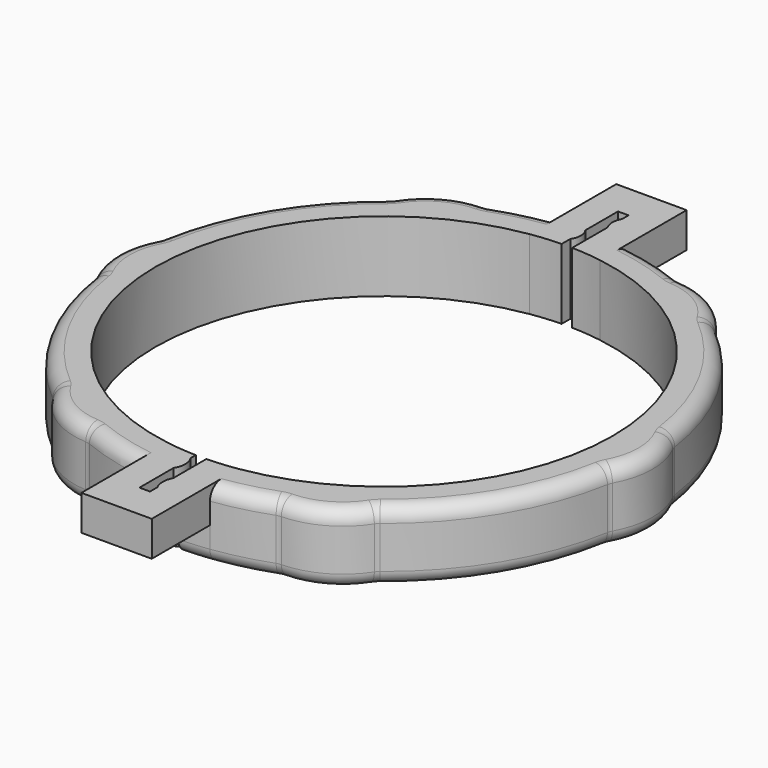
from build123d import *

# Parameters (mm, degrees)
F1_DEPTH = 10
F2_DEPTH = 5
F6_R     = 2


# Not quite as in the source:
# - a feature of the source that left no trace in its solid (it failed there, or was rolled back) is left out
# - the program builds the solid bodies; features that only make, move or delete a surface that nothing else refers to are left out


with BuildPart() as f1:
    # F0 (on Top) → F1 (new body)
    with BuildSketch(Plane.XY):
        with BuildLine():
            ThreePointArc((36.9932073794, -6.1443150788), (37.3730870863, -3.0825900858), (37.5, 0))
            ThreePointArc((37.5, 0), (37.4200494969, 2.4474263317), (37.1805388987, 4.8844167718))
            ThreePointArc((37.1805388987, 4.8844167718), (32.7897060145, 18.195746192), (23.8177366368, 28.9648998186))
            ThreePointArc((23.8177366368, 28.9648998186), (19.2988452952, 32.1528314503), (14.3602404423, 34.6414995986))
            ThreePointArc((14.3602404423, 34.6414995986), (9.762016079, 36.207085523), (5, 37.1651718683))
            Line((5, 37.1651718683), (5, 32.1130814467))
            ThreePointArc((5, 32.1130814467), (24.6855220727, 21.1394181566), (32.5, 0))
            ThreePointArc((32.5, 0), (24.6855220727, -21.1394181566), (5, -32.1130814467))
            Line((5, -32.1130814467), (5, -37.1651718683))
            ThreePointArc((5, -37.1651718683), (9.145691551, -36.367654943), (13.1754707426, -35.1092148974))
            ThreePointArc((13.1754707426, -35.1092148974), (18.195746192, -32.7897060145), (22.8202984564, -29.7570828268))
            ThreePointArc((22.8202984564, -29.7570828268), (32.1528314503, -19.2988452952), (36.9932073794, -6.1443150788))
        make_face()
        with BuildLine():
            ThreePointArc((37.1805388987, 4.8844167718), (37.4200494969, 2.4474263317), (37.5, 0))
            ThreePointArc((37.5, 0), (37.3730870863, -3.0825900858), (36.9932073794, -6.1443150788))
            ThreePointArc((36.9932073794, -6.1443150788), (38.5371895892, -0.6545838974), (37.1805388987, 4.8844167718))
        make_face()
        with BuildLine():
            ThreePointArc((14.3602404423, 34.6414995986), (19.2988452952, 32.1528314503), (23.8177366368, 28.9648998186))
            ThreePointArc((23.8177366368, 28.9648998186), (19.8354810786, 33.046893226), (14.3602404423, 34.6414995986))
        make_face()
        with BuildLine():
            ThreePointArc((13.1754707426, -35.1092148974), (18.7017085106, -33.7014771233), (22.8202984564, -29.7570828268))
            ThreePointArc((22.8202984564, -29.7570828268), (18.195746192, -32.7897060145), (13.1754707426, -35.1092148974))
        make_face()
        with BuildLine():
            Line((5, 32.1130814467), (5, 37.1651718683))
            ThreePointArc((5, 37.1651718683), (2.8796546327, 37.3892710439), (0.75, 37.4924992498))
            Line((0.75, 37.4924992498), (0.75, 32.4913450014))
            ThreePointArc((0.75, 32.4913450014), (2.8812142977, 32.3720342915), (5, 32.1130814467))
        make_face()
        with BuildLine():
            ThreePointArc((0.75, 37.4924992498), (2.8796546327, 37.3892710439), (5, 37.1651718683))
            Line((5, 37.1651718683), (5, 47.5))
            Line((5, 47.5), (-5, 47.5))
            Line((-5, 47.5), (-5, 37.1651718683))
            ThreePointArc((-5, 37.1651718683), (-2.8796546327, 37.3892710439), (-0.75, 37.4924992498))
            Line((-0.75, 37.4924992498), (-0.75, 42.5))
            Line((-0.75, 42.5), (0.75, 42.5))
            Line((0.75, 42.5), (0.75, 41.3848422468))
            ThreePointArc((0.75, 41.3848422468), (0.4052406825, 40.0777626783), (0.75, 38.7706831098))
            Line((0.75, 38.7706831098), (0.75, 37.4924992498))
        make_face()
        with BuildLine():
            Line((5, -47.5), (5, -37.1651718683))
            ThreePointArc((5, -37.1651718683), (2.8796546327, -37.3892710439), (0.75, -37.4924992498))
            Line((0.75, -37.4924992498), (0.75, -38.3779592812))
            ThreePointArc((0.75, -38.3779592812), (0.388658067, -39.7975817323), (0.75, -41.2172041833))
            Line((0.75, -41.2172041833), (0.75, -42.5))
            Line((0.75, -42.5), (-0.75, -42.5))
            Line((-0.75, -42.5), (-0.75, -37.4924992498))
            ThreePointArc((-0.75, -37.4924992498), (-2.8796546327, -37.3892710439), (-5, -37.1651718683))
            Line((-5, -37.1651718683), (-5, -47.5))
            Line((-5, -47.5), (5, -47.5))
        make_face()
        with BuildLine():
            ThreePointArc((0.75, -37.4924992498), (2.8796546327, -37.3892710439), (5, -37.1651718683))
            Line((5, -37.1651718683), (5, -32.1130814467))
            ThreePointArc((5, -32.1130814467), (2.8812142977, -32.3720342915), (0.75, -32.4913450014))
            Line((0.75, -32.4913450014), (0.75, -37.4924992498))
        make_face()
        with BuildLine():
            Line((-0.75, 36.7080494761), (-0.75, 37.4924992498))
            ThreePointArc((-0.75, 37.4924992498), (-2.8796546327, 37.3892710439), (-5, 37.1651718683))
            Line((-5, 37.1651718683), (-5, 32.1130814467))
            ThreePointArc((-5, 32.1130814467), (-2.8812142977, 32.3720342915), (-0.75, 32.4913450014))
            Line((-0.75, 32.4913450014), (-0.75, 34.0263359249))
            ThreePointArc((-0.75, 34.0263359249), (-0.3305926798, 35.3671927005), (-0.75, 36.7080494761))
        make_face()
        with BuildLine():
            ThreePointArc((-5, -37.1651718683), (-2.8796546327, -37.3892710439), (-0.75, -37.4924992498))
            Line((-0.75, -37.4924992498), (-0.75, -36.4494174719))
            ThreePointArc((-0.75, -36.4494174719), (-0.3154646596, -34.9226538092), (-0.75, -33.3958901465))
            Line((-0.75, -33.3958901465), (-0.75, -32.4913450014))
            ThreePointArc((-0.75, -32.4913450014), (-2.8812142977, -32.3720342915), (-5, -32.1130814467))
            Line((-5, -32.1130814467), (-5, -37.1651718683))
        make_face()
        with BuildLine():
            Line((-5, 32.1130814467), (-5, 37.1651718683))
            ThreePointArc((-5, 37.1651718683), (-9.145691551, 36.367654943), (-13.1754707426, 35.1092148974))
            ThreePointArc((-13.1754707426, 35.1092148974), (-18.195746192, 32.7897060145), (-22.8202984564, 29.7570828268))
            ThreePointArc((-22.8202984564, 29.7570828268), (-32.1528314503, 19.2988452952), (-36.9932073794, 6.1443150788))
            ThreePointArc((-36.9932073794, 6.1443150788), (-37.4945914872, 0.6368745642), (-37.1805388987, -4.8844167718))
            ThreePointArc((-37.1805388987, -4.8844167718), (-32.7897060145, -18.195746192), (-23.8177366368, -28.9648998186))
            ThreePointArc((-23.8177366368, -28.9648998186), (-19.2988452952, -32.1528314503), (-14.3602404423, -34.6414995986))
            ThreePointArc((-14.3602404423, -34.6414995986), (-9.762016079, -36.207085523), (-5, -37.1651718683))
            Line((-5, -37.1651718683), (-5, -32.1130814467))
            ThreePointArc((-5, -32.1130814467), (-32.5, 0), (-5, 32.1130814467))
        make_face()
        with BuildLine():
            ThreePointArc((-22.8202984564, 29.7570828268), (-18.195746192, 32.7897060145), (-13.1754707426, 35.1092148974))
            ThreePointArc((-13.1754707426, 35.1092148974), (-18.7017085106, 33.7014771233), (-22.8202984564, 29.7570828268))
        make_face()
        with BuildLine():
            ThreePointArc((-23.8177366368, -28.9648998186), (-19.8354810786, -33.046893226), (-14.3602404423, -34.6414995986))
            ThreePointArc((-14.3602404423, -34.6414995986), (-19.2988452952, -32.1528314503), (-23.8177366368, -28.9648998186))
        make_face()
        with BuildLine():
            ThreePointArc((-37.1805388987, -4.8844167718), (-37.4945914872, 0.6368745642), (-36.9932073794, 6.1443150788))
            ThreePointArc((-36.9932073794, 6.1443150788), (-38.5371895892, 0.6545838974), (-37.1805388987, -4.8844167718))
        make_face()
    extrude(amount=F1_DEPTH)

    # F0 (on Top) → F2 (cut)
    with BuildSketch(Plane.XY):
        with BuildLine():
            ThreePointArc((0.75, 37.4924992498), (2.8796546327, 37.3892710439), (5, 37.1651718683))
            Line((5, 37.1651718683), (5, 47.5))
            Line((5, 47.5), (-5, 47.5))
            Line((-5, 47.5), (-5, 37.1651718683))
            ThreePointArc((-5, 37.1651718683), (-2.8796546327, 37.3892710439), (-0.75, 37.4924992498))
            Line((-0.75, 37.4924992498), (-0.75, 42.5))
            Line((-0.75, 42.5), (0.75, 42.5))
            Line((0.75, 42.5), (0.75, 41.3848422468))
            ThreePointArc((0.75, 41.3848422468), (0.4052406825, 40.0777626783), (0.75, 38.7706831098))
            Line((0.75, 38.7706831098), (0.75, 37.4924992498))
        make_face()
        with BuildLine():
            Line((5, -47.5), (5, -37.1651718683))
            ThreePointArc((5, -37.1651718683), (2.8796546327, -37.3892710439), (0.75, -37.4924992498))
            Line((0.75, -37.4924992498), (0.75, -38.3779592812))
            ThreePointArc((0.75, -38.3779592812), (0.388658067, -39.7975817323), (0.75, -41.2172041833))
            Line((0.75, -41.2172041833), (0.75, -42.5))
            Line((0.75, -42.5), (-0.75, -42.5))
            Line((-0.75, -42.5), (-0.75, -37.4924992498))
            ThreePointArc((-0.75, -37.4924992498), (-2.8796546327, -37.3892710439), (-5, -37.1651718683))
            Line((-5, -37.1651718683), (-5, -47.5))
            Line((-5, -47.5), (5, -47.5))
        make_face()
    extrude(amount=F2_DEPTH, mode=Mode.SUBTRACT)

    # F6
    f6_edges = [f1.edges().sort_by_distance(p)[0] for p in [
        (-36.993207, 6.144315, 5),
        (-37.180539, -4.884417, 5),
        (-38.53719, 0.654584, 0),
        (-38.53719, 0.654584, 10),
        (-23.817737, -28.9649, 5),
        (-14.36024, -34.6415, 5),
        (-19.835481, -33.046893, 0),
        (-19.835481, -33.046893, 10),
        (-13.175471, 35.109215, 5),
        (-22.820298, 29.757083, 5),
        (-18.701709, 33.701477, 0),
        (-18.701709, 33.701477, 10),
        (23.817737, 28.9649, 5),
        (14.36024, 34.6415, 5),
        (19.835481, 33.046893, 0),
        (19.835481, 33.046893, 10),
        (36.993207, -6.144315, 5),
        (37.180539, 4.884417, 5),
        (38.53719, -0.654584, 0),
        (38.53719, -0.654584, 10),
        (13.175471, -35.109215, 5),
        (22.820298, -29.757083, 5),
        (18.701709, -33.701477, 0),
        (18.701709, -33.701477, 10),
        (9.145692, -36.367655, 10),
        (7.063972, -36.828661, 0),
        (-9.762016, -36.207086, 10),
        (-7.688426, -36.70338, 0),
        (-7.063972, 36.828661, 0),
        (-32.152831, 19.298845, 0),
        (-32.789706, -18.195746, 0),
        (-32.789706, -18.195746, 10),
        (-32.152831, 19.298845, 10),
        (-9.145692, 36.367655, 10),
        (9.762016, 36.207086, 10),
        (7.688426, 36.70338, 0),
        (32.789706, 18.195746, 0),
        (32.789706, 18.195746, 10),
        (32.152831, -19.298845, 0),
        (32.152831, -19.298845, 10),
    ]]
    fillet(f6_edges, radius=F6_R)


solid = f1.part
